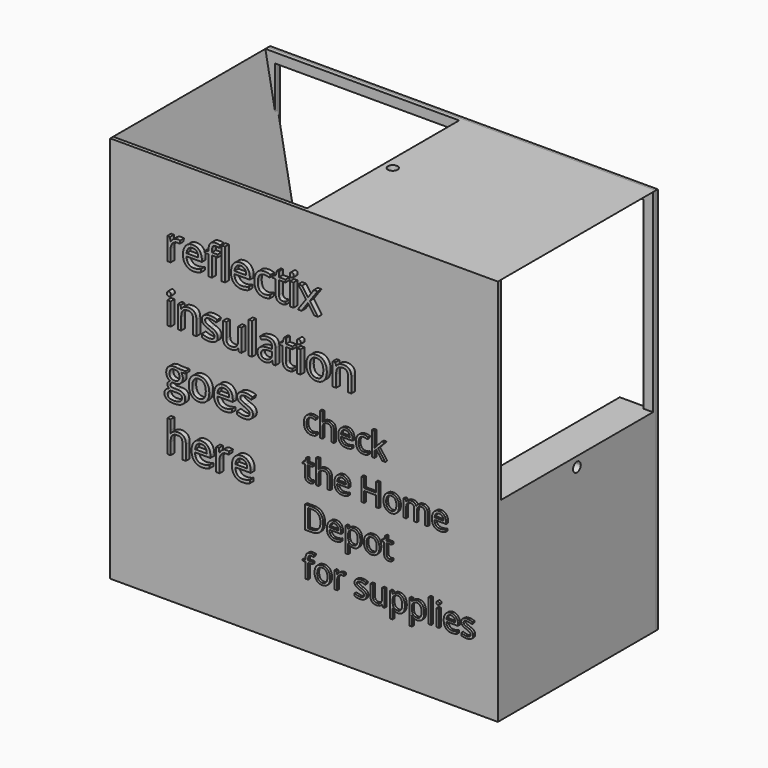
from build123d import *

# Parameters (mm, degrees)
F0_W         = 508
F0_H         = 508
F1_DEPTH     = 2.38125
F3_DEPTH     = 258.7625
F4_TEXT_SIZE = 54.5340693659
F5_DEPTH     = 6.35
F6_TEXT_SIZE = 41.3214787841
F7_DEPTH     = 3.175
F9_W         = 508
F9_H         = 508
F9_W_2       = 482.6
F9_H_2       = 482.6
F10_DEPTH    = 4.6355
F11_DEPTH    = 3.175
F13_R        = 6.35
F14_DEPTH    = 508.0010001
F15_R        = 6.35
F16_DEPTH    = 508.0010001
F18_DEPTH    = 508.0010001
F20_DEPTH    = 508.0010001


# Not quite as in the source:
# - Text() gives the source's letters only with a copy of the font that has no kerning and outlines rounded to 1/6400 em; it was checked with that copy


with BuildPart() as f1:
    # F0 (on Front) → F1 (new body, symmetric)
    with BuildSketch(Plane.XZ):
        Rectangle(F0_W, F0_H)
    extrude(amount=F1_DEPTH, both=True)

    # F2 (on face) → F3 (join)
    with BuildSketch(Plane.XZ.offset(2.38125)):
        Polygon((254, -254), (254, 0), (206.70520011, 0.0032258), align=None)
        Polygon((0, -206.6941250181), (-254, -254), (0, -254), align=None)
        Polygon((-206.6941250181, 0), (-254, 254), (-254, 0), align=None)
        Polygon((254, 254), (0, 254), (0, 206.6941250181), align=None)
    extrude(amount=-F3_DEPTH)

    # F4 (on face) → F5 (join)
    with BuildSketch(Plane.XZ.offset(2.38125)):
        with Locations((-178.8718104362, 140.853703022)):
            Text('reflectix', F4_TEXT_SIZE, font='Open Sans', text_align=(TextAlign.LEFT, TextAlign.BOTTOM))
        with Locations((-178.8718104362, 66.6873686843)):
            Text('insulation', F4_TEXT_SIZE, font='Open Sans', text_align=(TextAlign.LEFT, TextAlign.BOTTOM))
        with Locations((-178.8718104362, -7.4789656533)):
            Text('goes', F4_TEXT_SIZE, font='Open Sans', text_align=(TextAlign.LEFT, TextAlign.BOTTOM))
        with Locations((-178.8718104362, -81.645299991)):
            Text('here', F4_TEXT_SIZE, font='Open Sans', text_align=(TextAlign.LEFT, TextAlign.BOTTOM))
    extrude(amount=F5_DEPTH)

    # F6 (on face) → F7 (join)
    with BuildSketch(Plane.XZ.offset(2.38125)):
        with Locations((0, 0)):
            Text('check', F6_TEXT_SIZE, font='Open Sans', text_align=(TextAlign.LEFT, TextAlign.BOTTOM))
        with Locations((0, -56.1972111464)):
            Text('the Home', F6_TEXT_SIZE, font='Open Sans', text_align=(TextAlign.LEFT, TextAlign.BOTTOM))
        with Locations((0, -112.3944222927)):
            Text('Depot', F6_TEXT_SIZE, font='Open Sans', text_align=(TextAlign.LEFT, TextAlign.BOTTOM))
        with Locations((0, -168.5916334391)):
            Text('for supplies', F6_TEXT_SIZE, font='Open Sans', text_align=(TextAlign.LEFT, TextAlign.BOTTOM))
    extrude(amount=F7_DEPTH)


with BuildPart() as f10:
    # F9 (on offset) → F10 (new body)
    with BuildSketch(Plane.XZ.offset(-256.38125)):
        Rectangle(F9_W, F9_H)
        Rectangle(F9_W_2, F9_H_2, mode=Mode.SUBTRACT)
    extrude(amount=F10_DEPTH)


with BuildPart() as f11:
    # F11 (new): a face of the model
    f11_faces = [f10.part.faces().sort_by_distance(p)[0] for p in [
        (0, 256.38125, -246.8157951031),
    ]]
    extrude(f11_faces, amount=F11_DEPTH)


with BuildPart() as f10_1:
    add(f10.part)

    # F12: union F1
    add(f1.part)

    # F13 (on face) → F14 (cut, through all)
    with BuildSketch(Plane(origin=(-254, 0, 0), x_dir=(0, -1, 0), z_dir=(-1, 0, 0))):
        with Locations((-127.0635, 12.7)):
            Circle(F13_R)
    extrude(amount=-F14_DEPTH, mode=Mode.SUBTRACT)

    # F15 (on face) → F16 (cut, through all)
    with BuildSketch(Plane(origin=(0, 0, -254), x_dir=(1, 0, 0), z_dir=(0, 0, -1))):
        with Locations((-12.7, -123.0950504541)):
            Circle(F15_R)
    extrude(amount=-F16_DEPTH, mode=Mode.SUBTRACT)

    # F17 (on face) → F18 (cut, through all)
    with BuildSketch(Plane.YZ.offset(254)):
        with BuildLine():
            ThreePointArc((127.0635, -6.35), (122.5733719395, -17.1901280605), (133.4135, -12.7))
            ThreePointArc((133.4135, -12.7), (131.5536280605, -8.2098719395), (127.0635, -6.35))
        make_face()
    extrude(amount=-F18_DEPTH, mode=Mode.SUBTRACT)

    # F19 (on face) → F20 (cut, through all)
    with BuildSketch(Plane.XY.offset(254)):
        with BuildLine():
            ThreePointArc((19.05, 127.0635), (12.7, 133.4135), (6.35, 127.0635))
            ThreePointArc((6.35, 127.0635), (12.7, 120.7135), (19.05, 127.0635))
        make_face()
    extrude(amount=-F20_DEPTH, mode=Mode.SUBTRACT)


solid = Compound([f11.part, f10_1.part])
